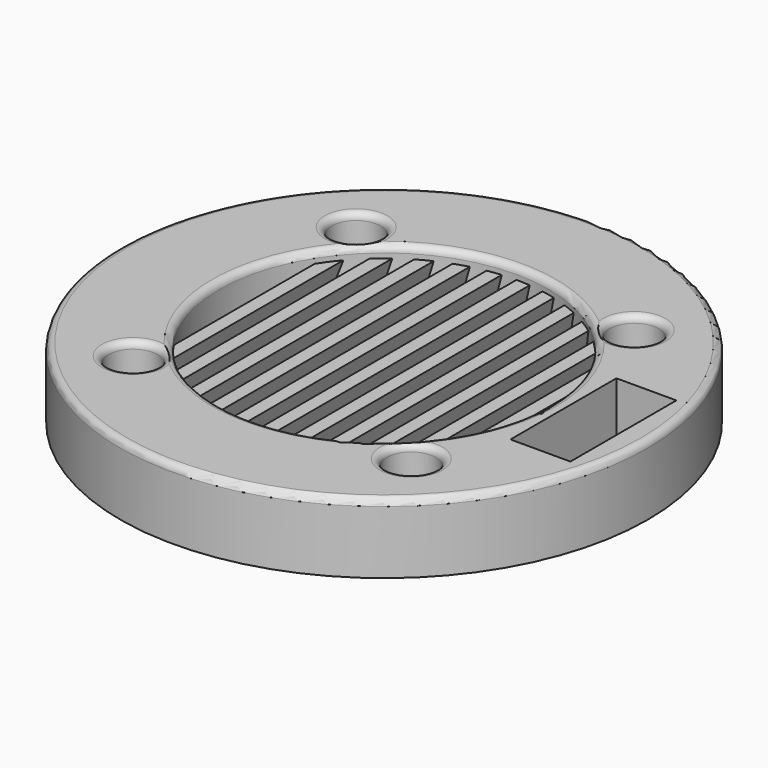
from build123d import *

# Parameters (mm, degrees)
F0_R      = 37.8107797269
F0_R_2    = 1.8255972752
F0_R_3    = 1.9467806804
F0_R_4    = 23.653060021
F0_W      = 8.5868872702
F0_H      = 18.9770264551
F0_R_5    = 1.8255985018
F1_DEPTH  = 10
F4_DEPTH  = 15.5
F5_DEPTH  = 19
F6_DEPTH  = 22
F7_DEPTH  = 24
F8_DEPTH  = 27.5
F9_DEPTH  = 27.5
F2_R      = 3.5
F2_R_2    = 1.8255985018
F2_R_3    = 1.8255972752
F2_R_4    = 1.9467806804
F10_DEPTH = 5


# Not quite as in the source:
# - a fillet or chamfer that OpenCascade refuses, or shapes differently, is made with other operations: its cross-section is extruded or revolved along the edge and cut away or added


with BuildPart() as f1:
    # F0 (on Top) → F1 (new body)
    with BuildSketch(Plane.XY):
        Circle(F0_R)
        with Locations((-19.9325345457, -20.0142711401)):
            Circle(F0_R_2, mode=Mode.SUBTRACT)
        with Locations((19.9106354266, -20.0142711401)):
            Circle(F0_R_2, mode=Mode.SUBTRACT)
        with Locations((-19.9325345457, 19.9147686362)):
            Circle(F0_R_3, mode=Mode.SUBTRACT)
        Circle(F0_R_4, mode=Mode.SUBTRACT)
        with Locations((29.9572963268, 0.0361171551)):
            Rectangle(F0_W, F0_H, mode=Mode.SUBTRACT)
        with Locations((19.9106372893, 19.9147686362)):
            Circle(F0_R_5, mode=Mode.SUBTRACT)
    extrude(amount=F1_DEPTH)

    # F3 (on Front) → F4 (join, symmetric)
    with BuildSketch(Plane.XZ):
        Polygon((-20.025298, 8.327912), (-22.067608, 0.072088), (-20.025298, 0.072088), (-18.055316, 8.327912), align=None)
        Polygon((20.097625, 8.327912), (18.055315, 0.072088), (20.097625, 0.072088), (22.067607, 8.327912), align=None)
    extrude(amount=F4_DEPTH, both=True)

    # F3 (on Front) → F5 (join, symmetric)
    with BuildSketch(Plane.XZ):
        Polygon((-16.013006, 8.327912), (-18.055316, 0.072088), (-16.013006, 0.072088), (-14.043023, 8.327912), align=None)
        Polygon((16.085333, 8.327912), (14.043023, 0.072088), (16.085333, 0.072088), (18.055315, 8.327912), align=None)
    extrude(amount=F5_DEPTH, both=True)

    # F3 (on Front) → F6 (join, symmetric)
    with BuildSketch(Plane.XZ):
        Polygon((-12.000714, 8.327912), (-14.043023, 0.072088), (-12.000714, 0.072088), (-10.030731, 8.327912), align=None)
        Polygon((12.07304, 8.327912), (10.03073, 0.072088), (12.07304, 0.072088), (14.043023, 8.327912), align=None)
    extrude(amount=F6_DEPTH, both=True)

    # F3 (on Front) → F7 (join, symmetric)
    with BuildSketch(Plane.XZ):
        Polygon((-7.988421, 8.327912), (-10.030731, 0.072088), (-7.988421, 0.072088), (-6.018439, 8.327912), align=None)
        Polygon((8.060748, 8.327912), (6.018438, 0.072088), (8.060748, 0.072088), (10.03073, 8.327912), align=None)
    extrude(amount=F7_DEPTH, both=True)

    # F3 (on Front) → F8 (join, symmetric)
    with BuildSketch(Plane.XZ):
        Polygon((-3.976129, 8.327912), (-6.018439, 0.072088), (-3.976129, 0.072088), (-2.006147, 8.327912), align=None)
        Polygon((4.048456, 8.327912), (2.006146, 0.072088), (4.048456, 0.072088), (6.018438, 8.327912), align=None)
    extrude(amount=F8_DEPTH, both=True)

    # F3 (on Front) → F9 (join, symmetric)
    with BuildSketch(Plane.XZ):
        Polygon((0.036163, 8.327912), (-2.006147, 0.072088), (0.036163, 0.072088), (2.006146, 8.327912), align=None)
    extrude(amount=F9_DEPTH, both=True)

    # F2 (on face) → F10 (cut)
    with BuildSketch(Plane.XY.offset(10)):
        with Locations((19.9106372893, 19.9147686362)):
            Circle(F2_R)
        with Locations((19.9106372893, 19.9147686362)):
            Circle(F2_R_2, mode=Mode.SUBTRACT)
        with Locations((-19.9325345457, -20.0142711401)):
            Circle(F2_R)
        with Locations((-19.9325345457, -20.0142711401)):
            Circle(F2_R_3, mode=Mode.SUBTRACT)
        with Locations((19.9106354266, -20.0142711401)):
            Circle(F2_R)
        with Locations((19.9106354266, -20.0142711401)):
            Circle(F2_R_3, mode=Mode.SUBTRACT)
        with Locations((-19.9325345457, 19.9147686362)):
            Circle(F2_R)
        with Locations((-19.9325345457, 19.9147686362)):
            Circle(F2_R_4, mode=Mode.SUBTRACT)
    extrude(amount=-F10_DEPTH, mode=Mode.SUBTRACT)

    # F11: fillet of radius 1 on 10 edges, made by hand

    # F11_s1 → F11_t2 (revolve, cut)
    with BuildSketch(Plane.XZ):
        with BuildLine():
            ThreePointArc((24.6540257064, 10.0004), (23.9459532398, 9.7071067812), (23.652660021, 8.9990343146))
            Line((23.652660021, 8.9990343146), (23.5525234525, 8.9990343146))
            ThreePointArc((23.5525234525, 8.9990343146), (23.5529234525, 9.4995171573), (23.5529234525, 10))
            Line((23.5529234525, 10), (23.653060021, 10.1001365685))
            ThreePointArc((23.653060021, 10.1001365685), (24.1535428637, 10.1001365685), (24.6540257064, 10.1005365685))
            Line((24.6540257064, 10.1005365685), (24.6540257064, 10.0004))
        make_face()
    revolve(axis=Axis((0, 0, 10), (0, 0, 1)), mode=Mode.SUBTRACT)

    # F11_s3 → F11_t4 (revolve, cut)
    with BuildSketch(Plane.XZ):
        with BuildLine():
            ThreePointArc((37.8111797269, 8.9990343146), (37.5178865081, 9.7071067812), (36.8098140415, 10.0004))
            Line((36.8098140415, 10.0004), (36.8098140415, 10.1005365685))
            ThreePointArc((36.8098140415, 10.1005365685), (37.3102968842, 10.1001365685), (37.8107797269, 10.1001365685))
            Line((37.8107797269, 10.1001365685), (37.9109162955, 10))
            ThreePointArc((37.9109162955, 10), (37.9109162955, 9.4995171573), (37.9113162955, 8.9990343146))
            Line((37.9113162955, 8.9990343146), (37.8111797269, 8.9990343146))
        make_face()
    revolve(axis=Axis((0, 0, 10), (0, 0, 1)), mode=Mode.SUBTRACT)

    # F11_s5 → F11_t6 (revolve, cut)
    with BuildSketch(Plane.XZ.offset(-19.9147686362)):
        with BuildLine():
            ThreePointArc((24.4116029747, 10.0004), (23.7035305081, 9.7071067812), (23.4102372893, 8.9990343146))
            Line((23.4102372893, 8.9990343146), (23.3101007207, 8.9990343146))
            ThreePointArc((23.3101007207, 8.9990343146), (23.3105007207, 9.4995171573), (23.3105007207, 10))
            Line((23.3105007207, 10), (23.4106372893, 10.1001365685))
            ThreePointArc((23.4106372893, 10.1001365685), (23.911120132, 10.1001365685), (24.4116029747, 10.1005365685))
            Line((24.4116029747, 10.1005365685), (24.4116029747, 10.0004))
        make_face()
    revolve(axis=Axis((19.9106372893, 19.9147686362, 10), (0, 0, 1)), mode=Mode.SUBTRACT)

    # F11_s7 → F11_t8 (revolve, cut)
    with BuildSketch(Plane.XZ.offset(20.0142711401)):
        with BuildLine():
            ThreePointArc((24.4116011121, 10.0004), (23.7035286455, 9.7071067812), (23.4102354266, 8.9990343146))
            Line((23.4102354266, 8.9990343146), (23.3100988581, 8.9990343146))
            ThreePointArc((23.3100988581, 8.9990343146), (23.3104988581, 9.4995171573), (23.3104988581, 10))
            Line((23.3104988581, 10), (23.4106354266, 10.1001365685))
            ThreePointArc((23.4106354266, 10.1001365685), (23.9111182694, 10.1001365685), (24.4116011121, 10.1005365685))
            Line((24.4116011121, 10.1005365685), (24.4116011121, 10.0004))
        make_face()
    revolve(axis=Axis((19.9106354266, -20.0142711401, 10), (0, 0, 1)), mode=Mode.SUBTRACT)

    # F11_s9 → F11_t10 (revolve, cut)
    with BuildSketch(Plane.XZ.offset(20.0142711401)):
        with BuildLine():
            ThreePointArc((-15.4315688602, 10.0004), (-16.1396413268, 9.7071067812), (-16.4329345457, 8.9990343146))
            Line((-16.4329345457, 8.9990343146), (-16.5330711142, 8.9990343146))
            ThreePointArc((-16.5330711142, 8.9990343146), (-16.5326711142, 9.4995171573), (-16.5326711142, 10))
            Line((-16.5326711142, 10), (-16.4325345457, 10.1001365685))
            ThreePointArc((-16.4325345457, 10.1001365685), (-15.9320517029, 10.1001365685), (-15.4315688602, 10.1005365685))
            Line((-15.4315688602, 10.1005365685), (-15.4315688602, 10.0004))
        make_face()
    revolve(axis=Axis((-19.9325345457, -20.0142711401, 10), (0, 0, 1)), mode=Mode.SUBTRACT)

    # F11_s11 → F11_t12 (revolve, cut)
    with BuildSketch(Plane.XZ.offset(-19.9147686362)):
        with BuildLine():
            ThreePointArc((-15.4315688602, 10.0004), (-16.1396413268, 9.7071067812), (-16.4329345457, 8.9990343146))
            Line((-16.4329345457, 8.9990343146), (-16.5330711142, 8.9990343146))
            ThreePointArc((-16.5330711142, 8.9990343146), (-16.5326711142, 9.4995171573), (-16.5326711142, 10))
            Line((-16.5326711142, 10), (-16.4325345457, 10.1001365685))
            ThreePointArc((-16.4325345457, 10.1001365685), (-15.9320517029, 10.1001365685), (-15.4315688602, 10.1005365685))
            Line((-15.4315688602, 10.1005365685), (-15.4315688602, 10.0004))
        make_face()
    revolve(axis=Axis((-19.9325345457, 19.9147686362, 10), (0, 0, 1)), mode=Mode.SUBTRACT)

    # F11_s13 → F11_t14 (revolve, cut)
    with BuildSketch(Plane.XZ.offset(-19.9147686362)):
        with BuildLine():
            ThreePointArc((-17.9861538653, 3.9990343146), (-17.6928606464, 4.7071067812), (-16.9847881798, 5.0004))
            Line((-16.9847881798, 5.0004), (-16.9847881798, 5.1005365685))
            ThreePointArc((-16.9847881798, 5.1005365685), (-17.4852710225, 5.1001365685), (-17.9857538653, 5.1001365685))
            Line((-17.9857538653, 5.1001365685), (-18.0858904338, 5))
            ThreePointArc((-18.0858904338, 5), (-18.0858904338, 4.4995171573), (-18.0862904338, 3.9990343146))
            Line((-18.0862904338, 3.9990343146), (-17.9861538653, 3.9990343146))
        make_face()
    revolve(axis=Axis((-19.9325345457, 19.9147686362, 5), (0, 0, 1)), mode=Mode.SUBTRACT)

    # F11_s15 → F11_t16 (revolve, cut)
    with BuildSketch(Plane.XZ.offset(20.0142711401)):
        with BuildLine():
            ThreePointArc((-18.1073372705, 3.9990343146), (-17.8140440516, 4.7071067812), (-17.105971585, 5.0004))
            Line((-17.105971585, 5.0004), (-17.105971585, 5.1005365685))
            ThreePointArc((-17.105971585, 5.1005365685), (-17.6064544278, 5.1001365685), (-18.1069372705, 5.1001365685))
            Line((-18.1069372705, 5.1001365685), (-18.207073839, 5))
            ThreePointArc((-18.207073839, 5), (-18.207073839, 4.4995171573), (-18.207473839, 3.9990343146))
            Line((-18.207473839, 3.9990343146), (-18.1073372705, 3.9990343146))
        make_face()
    revolve(axis=Axis((-19.9325345457, -20.0142711401, 5), (0, 0, 1)), mode=Mode.SUBTRACT)

    # F11_s17 → F11_t18 (revolve, cut)
    with BuildSketch(Plane.XZ.offset(20.0142711401)):
        with BuildLine():
            ThreePointArc((21.7358327018, 3.9990343146), (22.0291259207, 4.7071067812), (22.7371983873, 5.0004))
            Line((22.7371983873, 5.0004), (22.7371983873, 5.1005365685))
            ThreePointArc((22.7371983873, 5.1005365685), (22.2367155446, 5.1001365685), (21.7362327018, 5.1001365685))
            Line((21.7362327018, 5.1001365685), (21.6360961333, 5))
            ThreePointArc((21.6360961333, 5), (21.6360961333, 4.4995171573), (21.6356961333, 3.9990343146))
            Line((21.6356961333, 3.9990343146), (21.7358327018, 3.9990343146))
        make_face()
    revolve(axis=Axis((19.9106354266, -20.0142711401, 5), (0, 0, 1)), mode=Mode.SUBTRACT)

    # F11_s19 → F11_t20 (revolve, cut)
    with BuildSketch(Plane.XZ.offset(-19.9147686362)):
        with BuildLine():
            ThreePointArc((21.735835791, 3.9990343146), (22.0291290099, 4.7071067812), (22.7372014765, 5.0004))
            Line((22.7372014765, 5.0004), (22.7372014765, 5.1005365685))
            ThreePointArc((22.7372014765, 5.1005365685), (22.2367186338, 5.1001365685), (21.736235791, 5.1001365685))
            Line((21.736235791, 5.1001365685), (21.6360992225, 5))
            ThreePointArc((21.6360992225, 5), (21.6360992225, 4.4995171573), (21.6356992225, 3.9990343146))
            Line((21.6356992225, 3.9990343146), (21.735835791, 3.9990343146))
        make_face()
    revolve(axis=Axis((19.9106372893, 19.9147686362, 5), (0, 0, 1)), mode=Mode.SUBTRACT)


solid = f1.part
